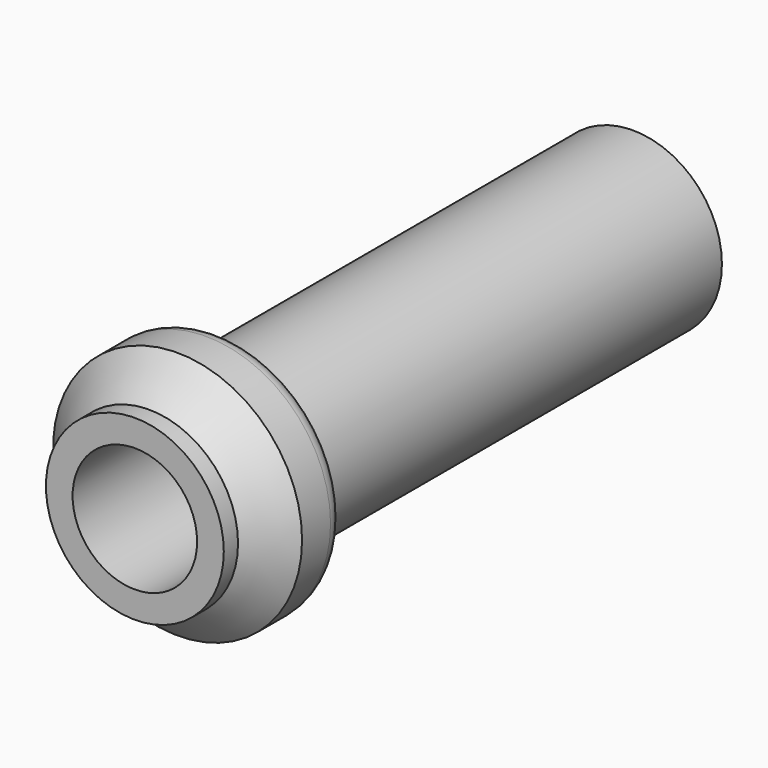
from build123d import *

# Parameters (mm, degrees)
F0_R     = 5
F0_R_2   = 3.5
F1_DEPTH = 35
F2_R     = 7
F2_R_2   = 5
F3_DEPTH = 6
F5_R     = 1


# Not quite as in the source:
# - a fillet or chamfer that OpenCascade refuses, or shapes differently, is made with other operations: its cross-section is extruded or revolved along the edge and cut away or added


with BuildPart() as f1:
    # F0 (on Front) → F1 (new body)
    with BuildSketch(Plane.XZ):
        Circle(F0_R)
        Circle(F0_R_2, mode=Mode.SUBTRACT)
    extrude(amount=F1_DEPTH)


with BuildPart() as f3:
    # F2 (on face) → F3 (new body)
    with BuildSketch(Plane.XZ.offset(35)):
        Circle(F2_R)
        Circle(F2_R_2, mode=Mode.SUBTRACT)
    extrude(amount=-F3_DEPTH)

    # F4: chamfer of 3 on 1 edges, made by hand

    # F4_s1 → F4_t2 (revolve, cut)
    with BuildSketch(Plane.XY):
        Polygon((7, -32), (4, -35), (7, -35), align=None)
    revolve(axis=Axis((0, -35, 0), (0, -1, 0)), mode=Mode.SUBTRACT)

    # F5
    f5_edges = [f3.edges().sort_by_distance(p)[0] for p in [
        (-7, -29, 0),
    ]]
    fillet(f5_edges, radius=F5_R)


solid = Compound([f1.part, f3.part])
